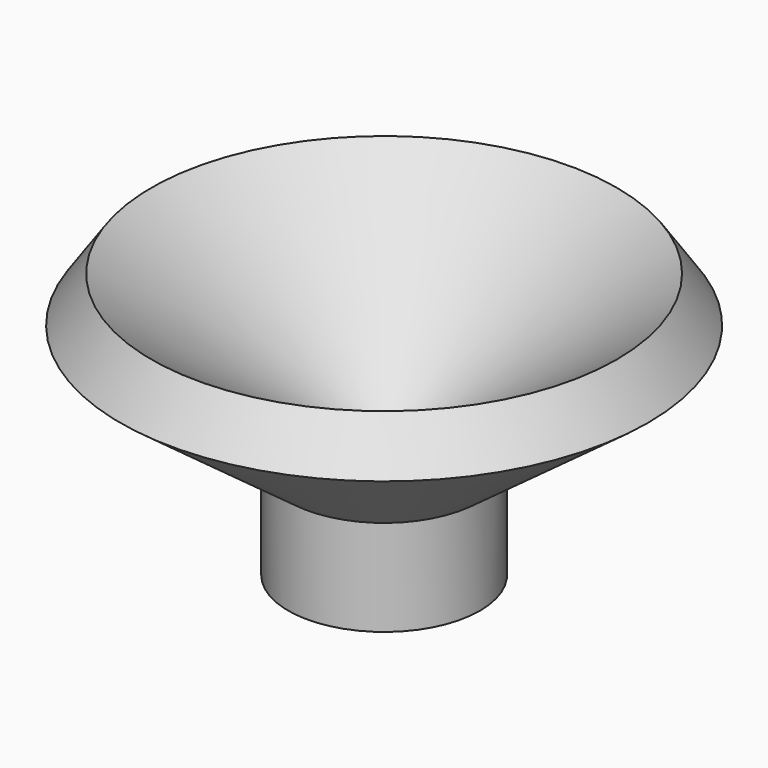
from build123d import *

# Parameters (mm, degrees)
F2_R     = 25.4
F3_DEPTH = 25.4
F4_DEPTH = 76.2


with BuildPart() as f1:
    # F0 (on Front) → F1 (revolve)
    with BuildSketch(Plane.XZ):
        Polygon((-58.1262356877, -14.8871221304), (-58.1262356877, -40.2871221304), (-32.7262356877, -40.2871221304), (-32.7262356877, -14.8871221304), (11.7363044992, 17.9430041462), (3.4545188379, 29.9932819682), align=None)
    revolve(axis=Axis((-58.1262356877, 0, -27.5871221304), (0, 0, -1)))


with BuildPart() as f3:
    # F2 (on face) → F3 (new body)
    with BuildSketch(Plane(origin=(0, 0, -40.2871221304), x_dir=(1, 0, 0), z_dir=(0, 0, -1))):
        with Locations((-58.1262356877, 0)):
            Circle(F2_R)
    extrude(amount=F3_DEPTH)

    # F4 (cut): a face of the model
    f4_faces = [f3.faces().sort_by_distance(p)[0] for p in [
        (-58.1262356877, 0, -65.6871221304),
    ]]
    extrude(f4_faces, amount=-F4_DEPTH, mode=Mode.SUBTRACT)


solid = f1.part
